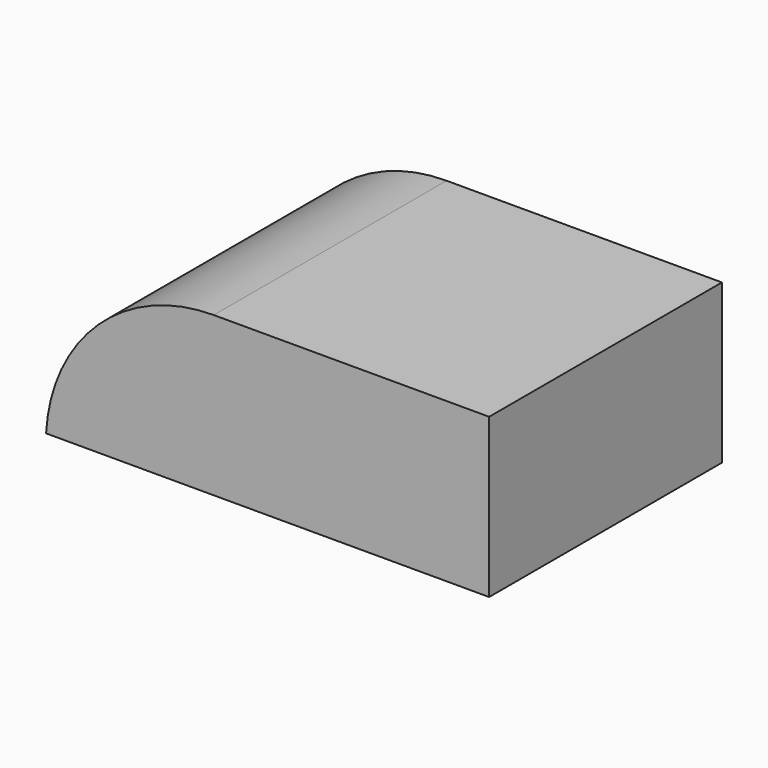
from build123d import *

# Parameters (mm, degrees)
F0_W        = 33.5
F0_H        = 22
F1_DEPTH    = 12
F2_T1_DEPTH = 85.4034699366


# Not quite as in the source:
# - a fillet or chamfer that OpenCascade refuses, or shapes differently, is made with other operations: its cross-section is extruded or revolved along the edge and cut away or added


with BuildPart() as f1:
    # F0 (on Top) → F1 (new body)
    with BuildSketch(Plane.XY):
        Rectangle(F0_W, F0_H)
    extrude(amount=F1_DEPTH)

    # F2: fillet of radius 12.7 on 1 edges, made by hand

    # F2_s2 → F2_t1 (cut)
    with BuildSketch(Plane.XZ.offset(-42.7017349683)):
        with BuildLine():
            ThreePointArc((-16.75, 0), (-12.7985671498, 8.5244241013), (-4.0693060127, 12))
            Line((-4.0693060127, 12), (-16.75, 12))
            Line((-16.75, 12), (-16.75, 0))
        make_face()
    extrude(amount=F2_T1_DEPTH, mode=Mode.SUBTRACT)


solid = f1.part
